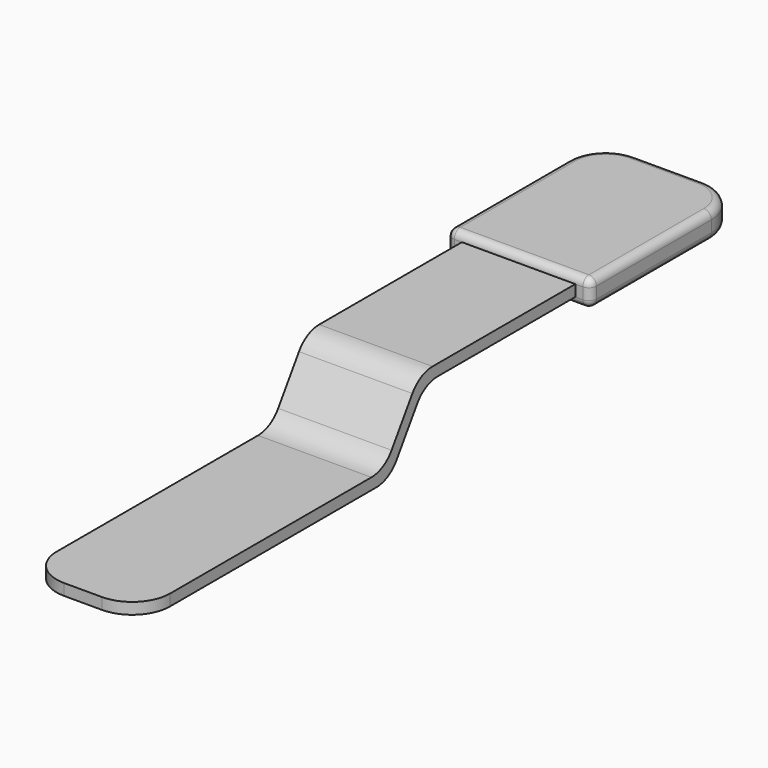
from build123d import *

# Parameters (mm, degrees)
F1_DEPTH = 15
F2_R     = 5
F3_W     = 19
F3_H     = 3.5
F4_DEPTH = 25
F5_R     = 5
F6_R     = 0.99999


# Not quite as in the source:
# - a fillet or chamfer is up to 0.001 mm smaller than in the source, because OpenCascade refuses the exact size


with BuildPart() as f1:
    # F0 (on Right) → F1 (new body)
    with BuildSketch(Plane.YZ):
        with BuildLine():
            Line((15.2185663986, 4.9061592609), (-8.3786299068, 4.9061592609))
            ThreePointArc((-8.3786299068, 4.9061592609), (-10.2743175345, 4.4284267718), (-11.7171893777, 3.10934347))
            Line((-11.7171893777, 3.10934347), (-15.1529792105, -2.0970249483))
            ThreePointArc((-15.1529792105, -2.0970249483), (-16.5958510537, -3.41610825), (-18.4915386814, -3.8938407391))
            Line((-18.4915386814, -3.8938407391), (-56.7814336014, -3.8938407391))
            Line((-56.7814336014, -3.8938407391), (-56.7814336014, -5.3938407391))
            Line((-56.7814336014, -5.3938407391), (-17.6842372959, -5.3938407391))
            ThreePointArc((-17.6842372959, -5.3938407391), (-15.7885496683, -4.91610825), (-14.3456778251, -3.5970249483))
            Line((-14.3456778251, -3.5970249483), (-10.9098879922, 1.60934347))
            ThreePointArc((-10.9098879922, 1.60934347), (-9.467016149, 2.9284267718), (-7.5713285214, 3.4061592609))
            Line((-7.5713285214, 3.4061592609), (15.2185663986, 3.4061592609))
            Line((15.2185663986, 3.4061592609), (15.2185663986, 4.9061592609))
        make_face()
    extrude(amount=-F1_DEPTH)

    # F2
    f2_edges = [f1.edges().sort_by_distance(p)[0] for p in [
        (-15, -56.781434, -4.643841),
        (0, -56.781434, -4.643841),
    ]]
    fillet(f2_edges, radius=F2_R)

    # F3 (on face) → F4 (join)
    with BuildSketch(Plane(origin=(0, 15.2185663986, 0), x_dir=(-1, 0, 0), z_dir=(0, 1, 0))):
        with Locations((7.5, 4.1561592609)):
            Rectangle(F3_W, F3_H)
    extrude(amount=F4_DEPTH)

    # F5
    f5_edges = [f1.edges().sort_by_distance(p)[0] for p in [
        (2, 40.218566, 4.156159),
        (-17, 40.218566, 4.156159),
    ]]
    fillet(f5_edges, radius=F5_R)

    # F6 (radius 1 in the source; OpenCascade refuses exactly that, so slightly less here)
    f6_edges = [f1.edges().sort_by_distance(p)[0] for p in [
        (-17, 25.218566, 5.906159),
        (-15.535534, 38.7541, 5.906159),
        (-7.5, 15.218566, 5.906159),
        (-7.5, 40.218566, 5.906159),
        (2, 25.218566, 5.906159),
        (0.535534, 38.7541, 5.906159),
        (2, 25.218566, 2.406159),
        (0.535534, 38.7541, 2.406159),
        (-7.5, 15.218566, 2.406159),
        (-7.5, 40.218566, 2.406159),
        (-17, 25.218566, 2.406159),
        (-15.535534, 38.7541, 2.406159),
        (2, 15.218566, 4.156159),
        (-17, 15.218566, 4.156159),
    ]]
    fillet(f6_edges, radius=F6_R)


solid = f1.part
